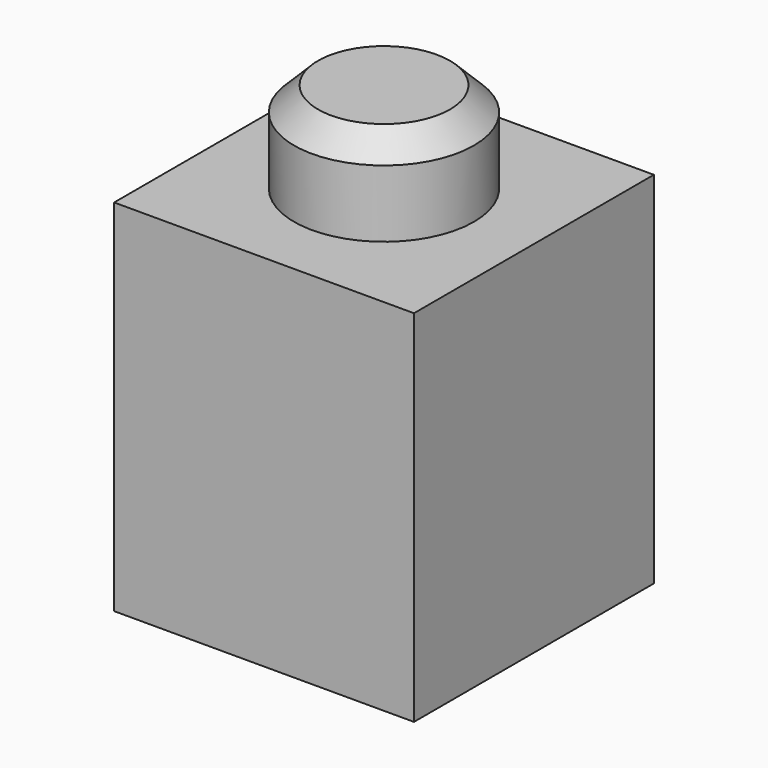
from build123d import *

# Parameters (mm, degrees)
F1_W     = 15.875
F1_H     = 19.05
F2_DEPTH = 7.9375
F3_R     = 4.7625
F4_DEPTH = 4.826
F5_SIZE  = 1.27
F6_T     = -1.5875


# Not quite as in the source:
# - a variable given as a bare number and used for a length is read in inches; the dataset says mm whatever the document's units were


with BuildPart() as f2:
    # F1 (on Front) → F2 (new body, symmetric)
    with BuildSketch(Plane.XZ):
        Rectangle(F1_W, F1_H)
    extrude(amount=F2_DEPTH, both=True)

    # F3 (on face) → F4 (join)
    with BuildSketch(Plane.XY.offset(9.525)):
        Circle(F3_R)
    extrude(amount=F4_DEPTH)

    # F5
    f5_edges = [f2.edges().sort_by_distance(p)[0] for p in [
        (-4.7625, 0, 14.351),
    ]]
    chamfer(f5_edges, length=F5_SIZE)

    # F6
    f6_openings = [f2.faces().sort_by_distance(p)[0] for p in [
        (0, 0, -9.525),
    ]]
    offset(amount=F6_T, openings=f6_openings, kind=Kind.INTERSECTION)


solid = f2.part
